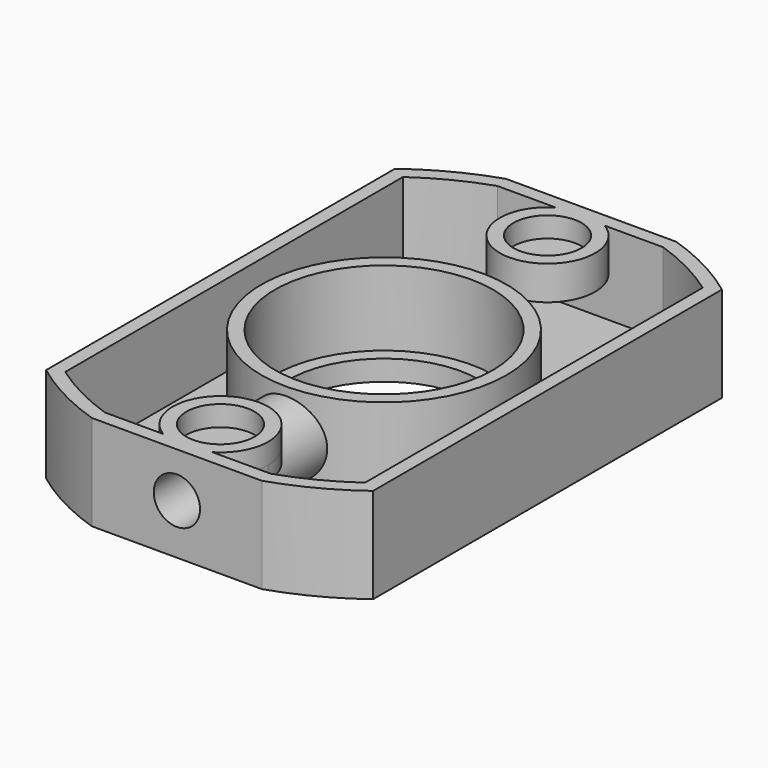
from build123d import *

# Parameters (mm, degrees)
F0_R     = 20
F0_R_2   = 7
F1_DEPTH = 7
F2_R     = 8
F3_DEPTH = 5.5
F4_R     = 2.5
F5_DEPTH = 1.5
F7_DEPTH = 25
F8_R     = 1.7
F9_DEPTH = 10
F10_T    = 1


# Not quite as in the source:
# - a shell that OpenCascade refuses in one call is made with other operations: the cavity is built on its own and cut out


with BuildPart() as f1:
    # F0 (on Top) → F1 (new body)
    with BuildSketch(Plane.XY):
        Circle(F0_R)
        Circle(F0_R_2, mode=Mode.SUBTRACT)
    extrude(amount=F1_DEPTH)

    # F2 (on face) → F3 (cut)
    with BuildSketch(Plane.XY.offset(7)):
        Circle(F2_R)
    extrude(amount=-F3_DEPTH, mode=Mode.SUBTRACT)

    # F4 (on face) → F5 (cut)
    with BuildSketch(Plane.XY.offset(7)):
        with Locations((0, 15)):
            Circle(F4_R)
        with Locations((0, -15)):
            Circle(F4_R)
    extrude(amount=-F5_DEPTH, mode=Mode.SUBTRACT)

    # F6 (on face) → F7 (cut)
    with BuildSketch(Plane.XY.offset(7)):
        with BuildLine():
            Line((-12, -16), (-12, 16))
            ThreePointArc((-12, 16), (-20, 0), (-12, -16))
        make_face()
        with BuildLine():
            Line((12, 16), (12, 19))
            Line((12, 19), (6.2449979984, 19))
            ThreePointArc((6.2449979984, 19), (9.2449979984, 17.7349939952), (12, 16))
        make_face()
        with BuildLine():
            ThreePointArc((-12, 16), (-9.2449979984, 17.7349939952), (-6.2449979984, 19))
            Line((-6.2449979984, 19), (-12, 19))
            Line((-12, 19), (-12, 16))
        make_face()
        with BuildLine():
            Line((12, -19), (12, -16))
            ThreePointArc((12, -16), (9.2449979984, -17.7349939952), (6.2449979984, -19))
            Line((6.2449979984, -19), (12, -19))
        make_face()
        with BuildLine():
            ThreePointArc((-6.2449979984, -19), (-9.2449979984, -17.7349939952), (-12, -16))
            Line((-12, -16), (-12, -19))
            Line((-12, -19), (-6.2449979984, -19))
        make_face()
        with BuildLine():
            ThreePointArc((20, 0), (17.88854382, 8.94427191), (12, 16))
            Line((12, 16), (12, -16))
            ThreePointArc((12, -16), (17.88854382, -8.94427191), (20, 0))
        make_face()
        with BuildLine():
            Line((-6.2449979984, 19), (6.2449979984, 19))
            ThreePointArc((6.2449979984, 19), (0, 20), (-6.2449979984, 19))
        make_face()
        with BuildLine():
            ThreePointArc((-6.2449979984, -19), (0, -20), (6.2449979984, -19))
            Line((6.2449979984, -19), (-6.2449979984, -19))
        make_face()
    extrude(amount=-F7_DEPTH, mode=Mode.SUBTRACT)

    # F8 (on face) → F9 (cut)
    with BuildSketch(Plane.XZ.offset(19)):
        with Locations((0, 3.6865652073)):
            Circle(F8_R)
    extrude(amount=-F9_DEPTH, mode=Mode.SUBTRACT)

    # F10: shell of thickness 1, made by hand


with BuildPart() as f10_core1:
    # F10_t2: copy of F1
    add(f1.part)

    # the walls: a layer under each face that stays
    f10_faces = [f10_core1.faces().sort_by_distance(p)[0] for p in [
        (9.2449979984, 17.7349939952, 3.5),
        (-8, -12.6666666667, 0),
        (0, 19, 3.5),
        (12, 0, 3.5),
        (9.2449979984, -17.7349939952, 3.5),
        (4.1633319989, -19, 1.1666666667),
        (-9.2449979984, -17.7349939952, 3.5),
        (-12, 0, 3.5),
        (-9.2449979984, 17.7349939952, 3.5),
        (-7, 0, 0.75),
        (-2.5, -15, 6.25),
        (-8, 0, 4.25),
        (-2.5, 15, 6.25),
        (-1.7, -14, 3.6865652073),
        (-5.3333333333, -5.3333333333, 1.5),
        (0, -15, 5.5),
        (0, 15, 5.5),
        (0, -9, 3.6865652073),
    ]]
    thicken(f10_faces, amount=-F10_T, mode=Mode.SUBTRACT)

    # F10_s3 → F10_t4 (revolve, cut)
    with BuildSketch(Plane.XZ.offset(15)):
        Polygon((2.49, 5.51), (3.5, 5.5), (3.5, 4.5), (2.5, 4.5), align=None)
    revolve(axis=Axis((0, -15, 5.5), (0, 0, 1)), mode=Mode.SUBTRACT)

    # F10_s5 → F10_t6 (revolve, cut)
    with BuildSketch(Plane.XZ):
        Polygon((7.99, 1.51), (9, 1.5), (9, 0.5), (8, 0.5), align=None)
    revolve(axis=Axis((0, 0, 1.5), (0, 0, 1)), mode=Mode.SUBTRACT)

    # F10_s7 → F10_t8 (revolve, cut)
    with BuildSketch(Plane.XZ.offset(-15)):
        Polygon((2.49, 5.51), (3.5, 5.5), (3.5, 4.5), (2.5, 4.5), align=None)
    revolve(axis=Axis((0, 15, 5.5), (0, 0, 1)), mode=Mode.SUBTRACT)

    # F10_s9 → F10_t10 (revolve, cut)
    with BuildSketch(Plane.XY.offset(3.6865652073)):
        Polygon((1.69, -9.01), (2.7, -9), (2.7, -8), (1.7, -8), align=None)
    revolve(axis=Axis((0, -9, 3.6865652073), (0, -1, 0)), mode=Mode.SUBTRACT)


with BuildPart() as f1_1:
    add(f1.part)

    # what is left inside the walls is the cavity
    f10_cavity = [f10_core1.part.solids().sort_by_distance(p)[0] for p in [
        (5.5, -14, 1.01),
    ]]
    add(f10_cavity, mode=Mode.SUBTRACT)


solid = f1_1.part
